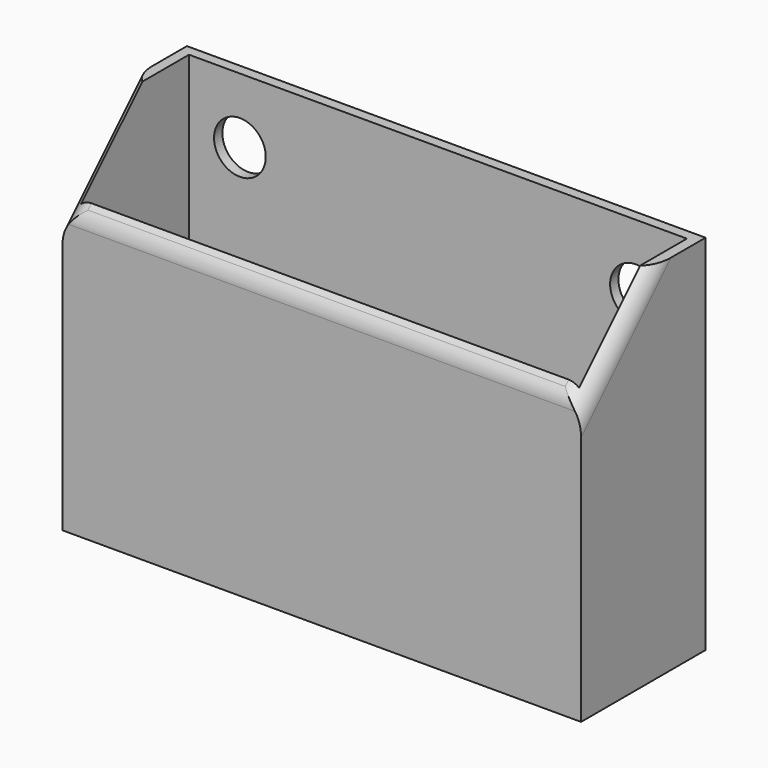
from build123d import *

# Parameters (mm, degrees)
F0_W        = 127
F0_H        = 88.9
F1_DEPTH    = 38.1
F2_T        = -2.54
F3_T1_DEPTH = 231.5131966309
F4_R        = 5.08
F5_R        = 6.333111045
F6_DEPTH    = 25.4


# Not quite as in the source:
# - a fillet or chamfer that OpenCascade refuses, or shapes differently, is made with other operations: its cross-section is extruded or revolved along the edge and cut away or added


with BuildPart() as f1:
    # F0 (on Front) → F1 (new body)
    with BuildSketch(Plane.XZ):
        Rectangle(F0_W, F0_H)
    extrude(amount=-F1_DEPTH)

    # F2
    f2_openings = [f1.faces().sort_by_distance(p)[0] for p in [
        (0, 19.05, 44.45),
    ]]
    offset(amount=F2_T, openings=f2_openings)

    # F3: chamfer of 20.32 on 1 edges, made by hand

    # F3_s2 → F3_t1 (cut)
    with BuildSketch(Plane.YZ.offset(-115.7565983155)):
        Polygon((0, 24.13), (20.32, 44.45), (0, 44.45), align=None)
    extrude(amount=F3_T1_DEPTH, mode=Mode.SUBTRACT)

    # F4
    f4_edges = [f1.edges().sort_by_distance(p)[0] for p in [
        (-63.5, 10.16, 34.29),
        (63.5, 10.16, 34.29),
        (0, 0, 24.13),
    ]]
    fillet(f4_edges, radius=F4_R)

    # F5 (on face) → F6 (cut)
    with BuildSketch(Plane(origin=(0, 38.1, 0), x_dir=(-1, 0, 0), z_dir=(0, 1, 0))):
        with Locations((-48.4922043979, 28.5164732486)):
            Circle(F5_R)
        with Locations((48.4922043979, 28.5164732486)):
            Circle(F5_R)
    extrude(amount=-F6_DEPTH, mode=Mode.SUBTRACT)


solid = f1.part
